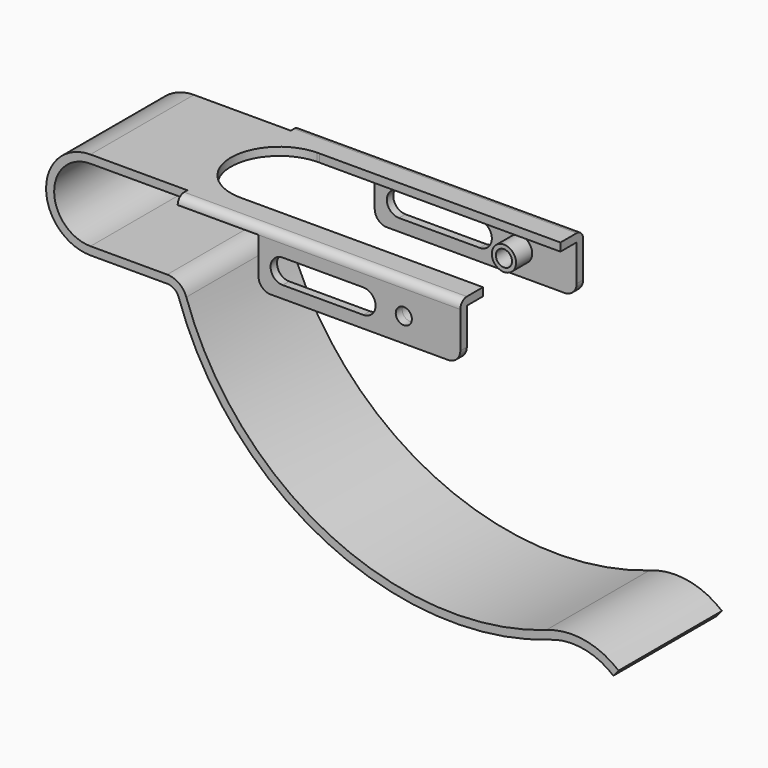
from build123d import *

# Parameters (mm, degrees)
F1_DEPTH  = 16
F2_W      = 70
F2_H      = 3
F3_DEPTH  = 2
F4_W      = 50
F4_H      = 14
F5_DEPTH  = 2
F6_R      = 2
F9_DEPTH  = 2
F11_DEPTH = 38.001
F13_D     = 4
F14_R     = 3
F14_R_2   = 2
F15_DEPTH = 5
F16_R     = 3


# Not quite as in the source:
# - a pattern or mirror of a feature is missing from the dataset's text; its kind, count and spacing are read off the source's solid


with BuildPart() as f1:
    # F0 (on Front) → F1 (new body)
    with BuildSketch(Plane.XZ):
        with BuildLine():
            ThreePointArc((0, -9), (-9, 0), (0, 9))
            Line((0, 9), (94, 9))
            Line((94, 9), (94, 11))
            Line((94, 11), (0, 11))
            ThreePointArc((0, 11), (-11, 0), (0, -11))
            Line((0, -11), (19, -11))
            ThreePointArc((19, -11), (20.7464347921, -11.5607448848), (21.84, -13.0333563221))
            ThreePointArc((21.84, -13.0333563221), (58.3659358906, -54.5122350868), (113.5320571839, -57.8797917247))
            ThreePointArc((113.5320571839, -57.8797917247), (121.8779484376, -57.0367571838), (129.5033807995, -60.5320954149))
            Line((129.5033807995, -60.5320954149), (130.788961497, -59))
            ThreePointArc((130.788961497, -59), (122.2254958147, -55.0670941025), (112.8483757943, -56))
            ThreePointArc((112.8483757943, -56), (59.2303979034, -52.7086373708), (23.7333333333, -12.3889272035))
            ThreePointArc((23.7333333333, -12.3889272035), (21.9107246536, -9.9345748081), (19, -9))
            Line((19, -9), (0, -9))
        make_face()
    extrude(amount=F1_DEPTH)

    # F2 (on face) → F3 (join)
    with BuildSketch(Plane.XY.offset(11)):
        with Locations((59, -17.5)):
            Rectangle(F2_W, F2_H)
    extrude(amount=-F3_DEPTH)

    # F4 (on face) → F5 (join)
    with BuildSketch(Plane.XZ.offset(19)):
        with Locations((69, 4)):
            Rectangle(F4_W, F4_H)
    extrude(amount=-F5_DEPTH)

    # F6
    f6_edges = [f1.edges().sort_by_distance(p)[0] for p in [
        (59, -19, 11),
    ]]
    fillet(f6_edges, radius=F6_R)

    # F7: F1 across plane


with BuildPart() as f1_1:
    add(f1.part)
    add(f1.part.mirror(Plane.XZ))

    # F8 (on face) → F9 (cut)
    with BuildSketch(Plane.XY.offset(11)):
        with BuildLine():
            Line((33.6929396674, 11.9960707714), (34.3070603326, 11.9960707714))
            ThreePointArc((34.3070603326, 11.9960707714), (34, 12), (33.6929396674, 11.9960707714))
        make_face()
        with BuildLine():
            Line((94, 11.9960707714), (34.3070603326, 11.9960707714))
            Line((34.3070603326, 11.9960707714), (33.6929396674, 11.9960707714))
            ThreePointArc((33.6929396674, 11.9960707714), (22.0074226206, -0.4220045025), (34.5369099172, -11.9879826385))
            Line((34.5369099172, -11.9879826385), (94, -11.9879826385))
            Line((94, -11.9879826385), (94, 11.9960707714))
        make_face()
    extrude(amount=-F9_DEPTH, mode=Mode.SUBTRACT)

    # F10 (on face) → F11 (cut, through all)
    with BuildSketch(Plane.XZ.offset(19)):
        with BuildLine():
            ThreePointArc((50, 6), (47, 3), (50, 0))
            Line((50, 0), (70, 0))
            ThreePointArc((70, 0), (73, 3), (70, 6))
            Line((70, 6), (50, 6))
        make_face()
    extrude(amount=-F11_DEPTH, mode=Mode.SUBTRACT)

    # F13 (through all)
    with Locations(Plane.XZ.offset(19)):
        with Locations((80, 3)):
            Hole(F13_D / 2)

    # F14 (on face) → F15 (join)
    with BuildSketch(Plane(origin=(0, -17, 0), x_dir=(-1, 0, 0), z_dir=(0, 1, 0))):
        with Locations((-80, 3)):
            Circle(F14_R)
        with Locations((-80, 3)):
            Circle(F14_R_2, mode=Mode.SUBTRACT)
    f15 = extrude(amount=F15_DEPTH)

    # F15_copies: F15 across plane
    add(f15.mirror(Plane.ZX))

    # F16
    f16_edges = [f1_1.edges().sort_by_distance(p)[0] for p in [
        (44, 18, -3),
        (44, -18, -3),
        (94, 18, -3),
        (94, -18, -3),
    ]]
    fillet(f16_edges, radius=F16_R)


solid = f1_1.part
